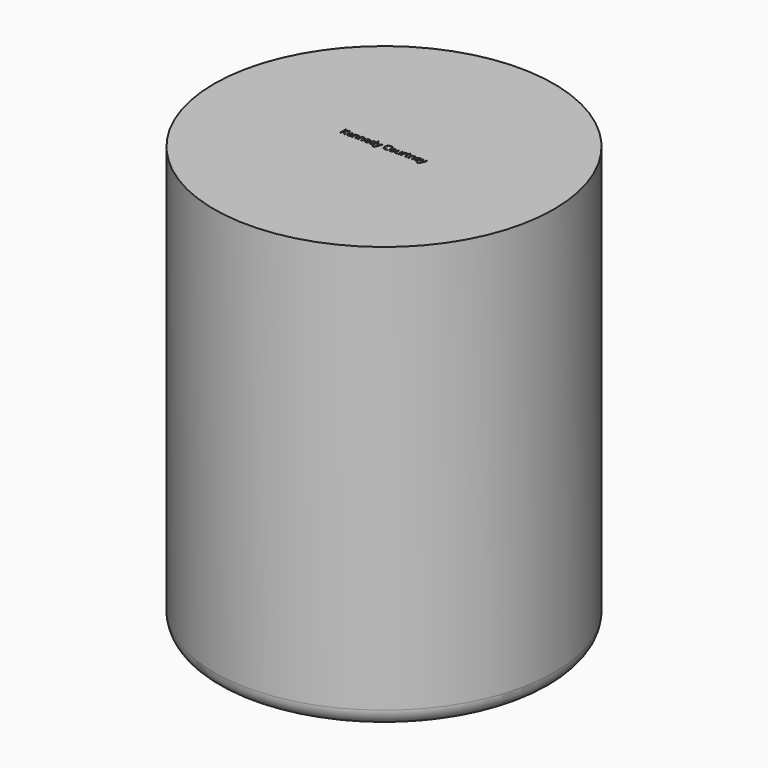
from build123d import *

# Parameters (mm, degrees)
F0_R         = 25.4
F1_DEPTH     = 2.54
F1_FACE_R    = 25.4
F2_DEPTH     = 63.5
F3_R         = 21.4882594132
F4_DEPTH     = 58.42
F5_R         = 2.54
F6_TEXT_SIZE = 1.4610033613
F7_DEPTH     = 0.5


# Not quite as in the source:
# - Text() gives the source's letters only with a copy of the font that has no kerning and outlines rounded to 1/6400 em; it was checked with that copy


with BuildPart() as f1:
    # F0 (on Top) → F1 (new body)
    with BuildSketch(Plane.XY):
        Circle(F0_R)
    extrude(amount=F1_DEPTH)

    # F0 (on Top) + F1_face (on face) → F2 (join)
    with BuildSketch(Plane.XY):
        Circle(F0_R)
    with BuildSketch(Plane(origin=(0, 0, 0), x_dir=(1, 0, 0), z_dir=(0, 0, -1))):
        Circle(F1_FACE_R)
    extrude(amount=F2_DEPTH, dir=(0, 0, 1))

    # F3 (on face) → F4 (cut)
    with BuildSketch(Plane(origin=(0, 0, 0), x_dir=(1, 0, 0), z_dir=(0, 0, -1))):
        Circle(F3_R)
    extrude(amount=-F4_DEPTH, mode=Mode.SUBTRACT)

    # F5
    f5_edges = [f1.edges().sort_by_distance(p)[0] for p in [
        (-25.4, 0, 0),
    ]]
    fillet(f5_edges, radius=F5_R)

    # F6 (on face) → F7 (cut)
    with BuildSketch(Plane.XY.offset(63.5)):
        with Locations((-6.35, -0.4552397664)):
            Text('Kennedy Courtney', F6_TEXT_SIZE, font='Open Sans', text_align=(TextAlign.LEFT, TextAlign.BOTTOM))
    extrude(amount=-F7_DEPTH, mode=Mode.SUBTRACT)


solid = f1.part
